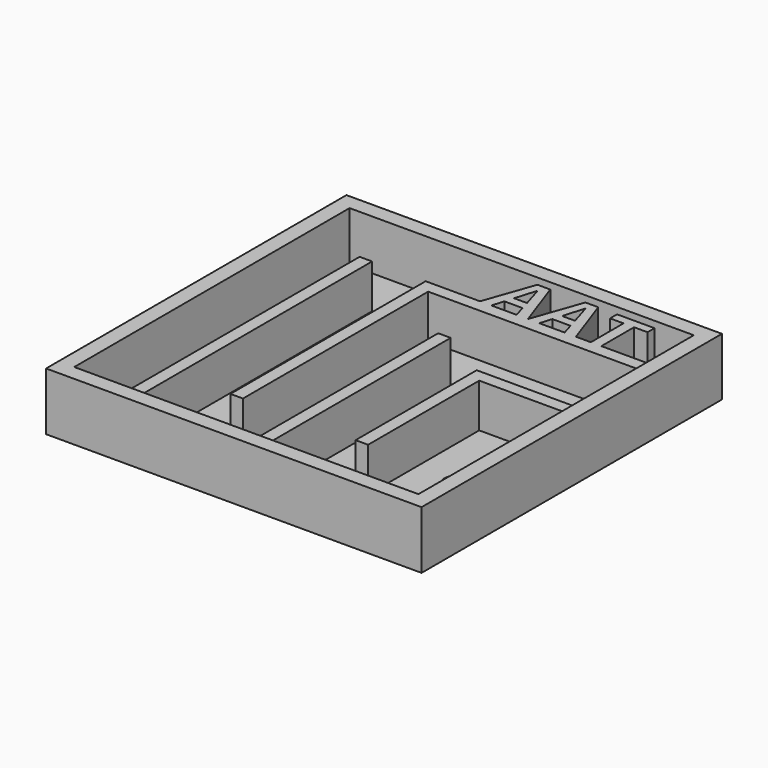
from build123d import *

# Parameters (mm, degrees)
F0_W         = 38.1
F0_H         = 38.1
F1_DEPTH     = 0.79375
F2_W         = 38.1
F2_H         = 38.1
F2_W_2       = 34.925
F2_H_2       = 34.925
F3_DEPTH     = 5.08
F4_W         = 1.27
F4_H         = 23.495
F4_H_2       = 29.845
F4_TEXT_SIZE = 7.0555555556
F5_DEPTH     = 4.445
F6_R         = 1.27
F7_DEPTH     = 0.0396875


# Not quite as in the source:
# - Text() gives the source's letters only with a copy of the font that has no kerning and outlines rounded to 1/6400 em; it was checked with that copy


with BuildPart() as f1:
    # F0 (on Top) → F1 (new body)
    with BuildSketch(Plane.XY):
        with Locations((2.1393038332, 0.0917097063)):
            Rectangle(F0_W, F0_H)
    extrude(amount=F1_DEPTH)

    # F2 (on face) → F3 (join)
    with BuildSketch(Plane.XY.offset(0.79375)):
        with Locations((2.1393038332, 0.0917097063)):
            Rectangle(F2_W, F2_H)
        with Locations((2.1393038332, 0.0917097063)):
            Rectangle(F2_W_2, F2_H_2, mode=Mode.SUBTRACT)
    extrude(amount=F3_DEPTH)

    # F4 (on face) → F5 (join)
    with BuildSketch(Plane.XY.offset(0.79375)):
        with Locations((3.4460787574, -5.6232902937)):
            Rectangle(F4_W, F4_H)
        Polygon((10.4310787574, 1.8042636802), (19.6018038332, 1.8042636802), (19.6018038332, 3.0742636802), (10.4310787574, 3.0742636802), (9.1610787574, 3.0742636802), (9.1610787574, 1.8042636802), (9.1610787574, -12.2907902937), (10.4310787574, -12.2907902937), align=None)
        Polygon((19.6018038332, 11.2042097063), (19.6018038332, 12.4742097063), (14.2890777365, 12.4742097063), (13.2208225282, 12.4742097063), (11.7115950976, 12.4742097063), (10.5606575976, 12.4742097063), (7.9941992643, 12.4742097063), (6.8432617643, 12.4742097063), (5.6923242643, 12.4742097063), (3.1258659309, 12.4742097063), (1.9749284309, 12.4742097063), (-2.2689212426, 12.4742097063), (-3.5389212426, 12.4742097063), (-3.5389212426, 11.2042097063), (-3.5389212426, -12.2907902937), (-2.2689212426, -12.2907902937), (-2.2689212426, 11.2042097063), align=None)
        with Locations((-9.6081961668, -2.4482902937)):
            Rectangle(F4_W, F4_H_2)
        with Locations((1.9749284309, 12.4742097063)):
            Text('AAT', F4_TEXT_SIZE, font='Open Sans', font_style=FontStyle.BOLD, text_align=(TextAlign.LEFT, TextAlign.BOTTOM))
    extrude(amount=F5_DEPTH)

    # F6 (on face) → F7 (cut)
    with BuildSketch(Plane.XY.offset(0.79375)):
        with Locations((-12.7831961668, -13.5607902937)):
            Circle(F6_R)
        with Locations((14.6734397858, -6.3466643915)):
            Circle(F6_R)
    extrude(amount=-F7_DEPTH, mode=Mode.SUBTRACT)


solid = f1.part
